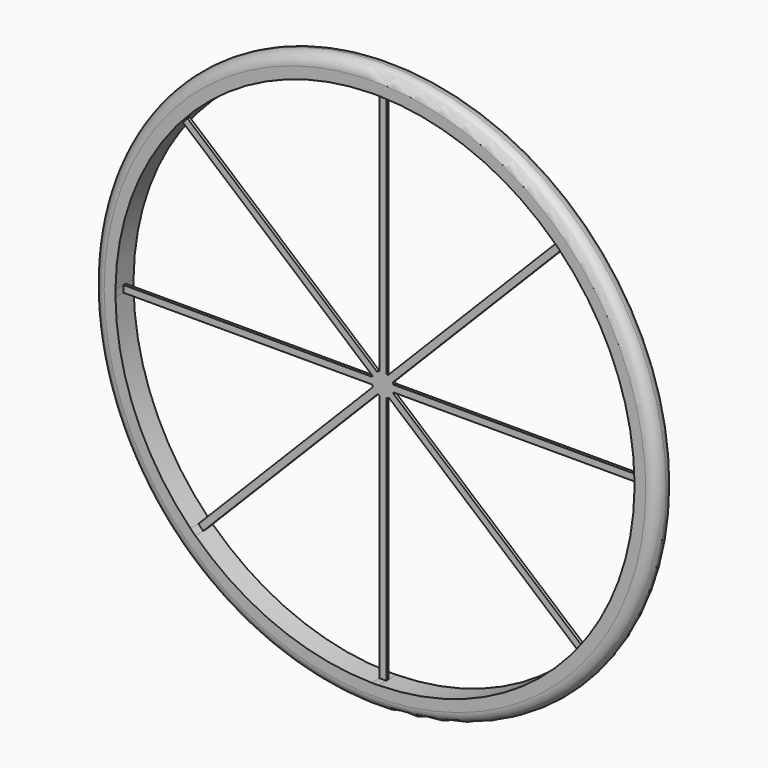
from build123d import *

# Parameters (mm, degrees)
F0_R     = 317.5
F1_DEPTH = 12.7
F2_DEPTH = 1.5875
F3_R     = 12.69999


# Not quite as in the source:
# - a fillet or chamfer is up to 0.001 mm smaller than in the source, because OpenCascade refuses the exact size


with BuildPart() as f1:
    # F0 (on Front) → F1 (new body, symmetric)
    with BuildSketch(Plane.XZ):
        Circle(F0_R)
        with BuildLine():
            ThreePointArc((207.6362893124, 205.4497051849), (269.4299975889, 112.8267982318), (292.075151117, 3.81))
            ThreePointArc((292.075151117, 3.81), (292.0937877132, 1.9050405158), (292.1, 0))
            ThreePointArc((292.1, 0), (292.0937877132, -1.9050405158), (292.075151117, -3.81))
            ThreePointArc((292.075151117, -3.81), (274.1141878064, -100.9149247795), (224.8232220619, -186.4857335607))
            ThreePointArc((224.8232220619, -186.4857335607), (222.371673788, -189.4023460697), (219.8822912949, -192.2867337465))
            ThreePointArc((219.8822912949, -192.2867337465), (122.4703733828, -265.1856286519), (3.81, -292.075151117))
            ThreePointArc((3.81, -292.075151117), (0, -292.1), (-3.81, -292.075151117))
            ThreePointArc((-3.81, -292.075151117), (-110.7351842209, -270.2963724795), (-202.2065364328, -210.7959359756))
            ThreePointArc((-202.2065364328, -210.7959359756), (-204.9388469754, -208.1405270493), (-207.6362893124, -205.4497051849))
            ThreePointArc((-207.6362893124, -205.4497051849), (-269.4299975889, -112.8267982318), (-292.075151117, -3.81))
            ThreePointArc((-292.075151117, -3.81), (-292.1, 0), (-292.075151117, 3.81))
            ThreePointArc((-292.075151117, 3.81), (-274.1141878064, 100.9149247795), (-224.8232220619, 186.4857335607))
            ThreePointArc((-224.8232220619, 186.4857335607), (-222.371673788, 189.4023460697), (-219.8822912949, 192.2867337465))
            ThreePointArc((-219.8822912949, 192.2867337465), (-122.4703733828, 265.1856286519), (-3.81, 292.075151117))
            ThreePointArc((-3.81, 292.075151117), (0, 292.1), (3.81, 292.075151117))
            ThreePointArc((3.81, 292.075151117), (110.7351842209, 270.2963724795), (202.2065364328, 210.7959359756))
            ThreePointArc((202.2065364328, 210.7959359756), (204.9388469754, 208.1405270493), (207.6362893124, 205.4497051849))
        make_face(mode=Mode.SUBTRACT)
    extrude(amount=F1_DEPTH, both=True)

    # F0 (on Front) → F2 (join, symmetric)
    with BuildSketch(Plane.XZ):
        with BuildLine():
            ThreePointArc((-3.81, 12.115027858), (0, 12.7), (3.81, 12.115027858))
            Line((3.81, 12.115027858), (3.81, 292.075151117))
            ThreePointArc((3.81, 292.075151117), (0, 292.1), (-3.81, 292.075151117))
            Line((-3.81, 292.075151117), (-3.81, 12.115027858))
        make_face()
        with BuildLine():
            ThreePointArc((-11.6934678579, 4.9550791574), (-9.668333643, 8.2348846117), (-6.7525370909, 10.7560793432))
            Line((-6.7525370909, 10.7560793432), (-219.8822912949, 192.2867337465))
            ThreePointArc((-219.8822912949, 192.2867337465), (-222.371673788, 189.4023460697), (-224.8232220619, 186.4857335607))
            Line((-224.8232220619, 186.4857335607), (-11.6934678579, 4.9550791574))
        make_face()
        with BuildLine():
            ThreePointArc((5.7850887786, 11.3058722717), (8.9103846511, 9.0495881326), (11.2148416582, 5.959641481))
            Line((11.2148416582, 5.959641481), (207.6362893124, 205.4497051849))
            ThreePointArc((207.6362893124, 205.4497051849), (204.9388469754, 208.1405270493), (202.2065364328, 210.7959359756))
            Line((202.2065364328, 210.7959359756), (5.7850887786, 11.3058722717))
        make_face()
        with BuildLine():
            ThreePointArc((12.115027858, 3.81), (12.5529051179, 1.9273227809), (12.7, 0))
            ThreePointArc((12.7, 0), (12.5529051179, -1.9273227809), (12.115027858, -3.81))
            Line((12.115027858, -3.81), (292.075151117, -3.81))
            ThreePointArc((292.075151117, -3.81), (292.0937877132, -1.9050405158), (292.1, 0))
            ThreePointArc((292.1, 0), (292.0937877132, 1.9050405158), (292.075151117, 3.81))
            Line((292.075151117, 3.81), (12.115027858, 3.81))
        make_face()
        with BuildLine():
            Line((224.8232220619, -186.4857335607), (11.6934678579, -4.9550791574))
            ThreePointArc((11.6934678579, -4.9550791574), (9.668333643, -8.2348846117), (6.7525370909, -10.7560793432))
            Line((6.7525370909, -10.7560793432), (219.8822912949, -192.2867337465))
            ThreePointArc((219.8822912949, -192.2867337465), (222.371673788, -189.4023460697), (224.8232220619, -186.4857335607))
        make_face()
        with BuildLine():
            Line((3.81, -292.075151117), (3.81, -12.115027858))
            ThreePointArc((3.81, -12.115027858), (0, -12.7), (-3.81, -12.115027858))
            Line((-3.81, -12.115027858), (-3.81, -292.075151117))
            ThreePointArc((-3.81, -292.075151117), (0, -292.1), (3.81, -292.075151117))
        make_face()
        with BuildLine():
            ThreePointArc((-12.115027858, -3.81), (-12.7, 0), (-12.115027858, 3.81))
            Line((-12.115027858, 3.81), (-292.075151117, 3.81))
            ThreePointArc((-292.075151117, 3.81), (-292.1, 0), (-292.075151117, -3.81))
            Line((-292.075151117, -3.81), (-12.115027858, -3.81))
        make_face()
        with BuildLine():
            Line((-202.2065364328, -210.7959359756), (-5.7850887786, -11.3058722717))
            ThreePointArc((-5.7850887786, -11.3058722717), (-8.9103846511, -9.0495881326), (-11.2148416582, -5.959641481))
            Line((-11.2148416582, -5.959641481), (-207.6362893124, -205.4497051849))
            ThreePointArc((-207.6362893124, -205.4497051849), (-204.9388469754, -208.1405270493), (-202.2065364328, -210.7959359756))
        make_face()
        with BuildLine():
            ThreePointArc((12.115027858, -3.81), (12.5529051179, -1.9273227809), (12.7, 0))
            ThreePointArc((12.7, 0), (12.5529051179, 1.9273227809), (12.115027858, 3.81))
            ThreePointArc((12.115027858, 3.81), (11.7143477213, 4.9055129666), (11.2148416582, 5.959641481))
            ThreePointArc((11.2148416582, 5.959641481), (8.9103846511, 9.0495881326), (5.7850887786, 11.3058722717))
            ThreePointArc((5.7850887786, 11.3058722717), (4.814573227, 11.7520161948), (3.81, 12.115027858))
            ThreePointArc((3.81, 12.115027858), (0, 12.7), (-3.81, 12.115027858))
            ThreePointArc((-3.81, 12.115027858), (-5.3247988427, 11.5298099414), (-6.7525370909, 10.7560793432))
            ThreePointArc((-6.7525370909, 10.7560793432), (-9.668333643, 8.2348846117), (-11.6934678579, 4.9550791574))
            ThreePointArc((-11.6934678579, 4.9550791574), (-11.9180081655, 4.3876054252), (-12.115027858, 3.81))
            ThreePointArc((-12.115027858, 3.81), (-12.7, 0), (-12.115027858, -3.81))
            ThreePointArc((-12.115027858, -3.81), (-11.7143477213, -4.9055129666), (-11.2148416582, -5.959641481))
            ThreePointArc((-11.2148416582, -5.959641481), (-8.9103846511, -9.0495881326), (-5.7850887786, -11.3058722717))
            ThreePointArc((-5.7850887786, -11.3058722717), (-4.814573227, -11.7520161948), (-3.81, -12.115027858))
            ThreePointArc((-3.81, -12.115027858), (0, -12.7), (3.81, -12.115027858))
            ThreePointArc((3.81, -12.115027858), (5.3247988427, -11.5298099414), (6.7525370909, -10.7560793432))
            ThreePointArc((6.7525370909, -10.7560793432), (9.668333643, -8.2348846117), (11.6934678579, -4.9550791574))
            ThreePointArc((11.6934678579, -4.9550791574), (11.9180081655, -4.3876054252), (12.115027858, -3.81))
        make_face()
    extrude(amount=F2_DEPTH, both=True)

    # F3 (radius 12.7 in the source; OpenCascade refuses exactly that, so slightly less here)
    f3_edges = [f1.edges().sort_by_distance(p)[0] for p in [
        (-317.5, -12.7, 0),
        (-317.5, 12.7, 0),
    ]]
    fillet(f3_edges, radius=F3_R)


solid = f1.part
